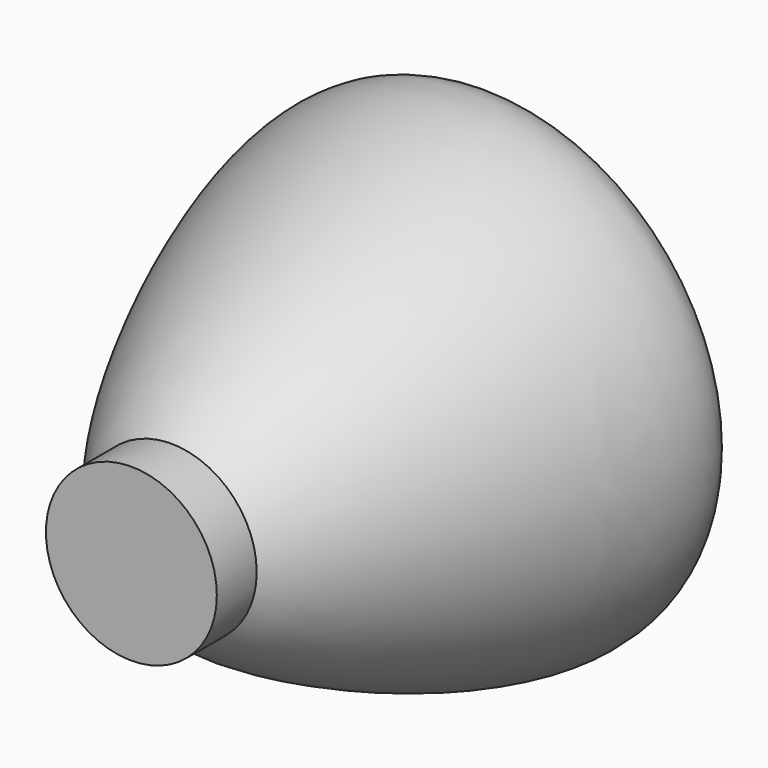
from build123d import *


with BuildPart() as f1:
    # F0 (on Top) → F1 (revolve)
    with BuildSketch(Plane.XY):
        with BuildLine():
            Line((10.4394918308, -25.5203954875), (0, -25.5203954875))
            Line((0, -25.5203954875), (0, -28.1940009445))
            Line((0, -28.1940009445), (10.9728025272, -28.1940009445))
            add(Edge.make_bspline(
                [(10.9728025272, -28.1940009445), (21.1413321645, -18.8934123486), (35.8877876093, 15.5730034128), (30.4799992591, 22.0980010927)],
                knots=[0.3901033008, 0.3901033008, 0.3901033008, 0.3901033008, 0.7223966542, 0.7223966542, 0.7223966542, 0.7223966542], degree=3))
            Line((30.4799992591, 22.0980010927), (10.4394918308, -25.5203954875))
        make_face()
        with BuildLine():
            add(Edge.make_bspline(
                [(0, -28.1940009445), (2.7316766907, -31.4643099771), (6.3866282791, -32.388719496), (10.9728025272, -28.1940009445)],
                knots=[0.2402335286, 0.2402335286, 0.2402335286, 0.2402335286, 0.3901033008, 0.3901033008, 0.3901033008, 0.3901033008], degree=3))
            Line((0, -28.1940009445), (0, -34.5948003232))
            Line((0, -34.5948003232), (10.9728025272, -34.5948003232))
            Line((10.9728025272, -34.5948003232), (10.9728025272, -28.1940009445))
        make_face()
        with BuildLine():
            Line((10.9728025272, -28.1940009445), (0, -28.1940009445))
            add(Edge.make_bspline(
                [(0, -28.1940009445), (2.7316766907, -31.4643099771), (6.3866282791, -32.388719496), (10.9728025272, -28.1940009445)],
                knots=[0.2402335286, 0.2402335286, 0.2402335286, 0.2402335286, 0.3901033008, 0.3901033008, 0.3901033008, 0.3901033008], degree=3))
        make_face()
    revolve(axis=Axis((0, -1.0668002069, 0), (0, -1, 0)))


solid = f1.part
